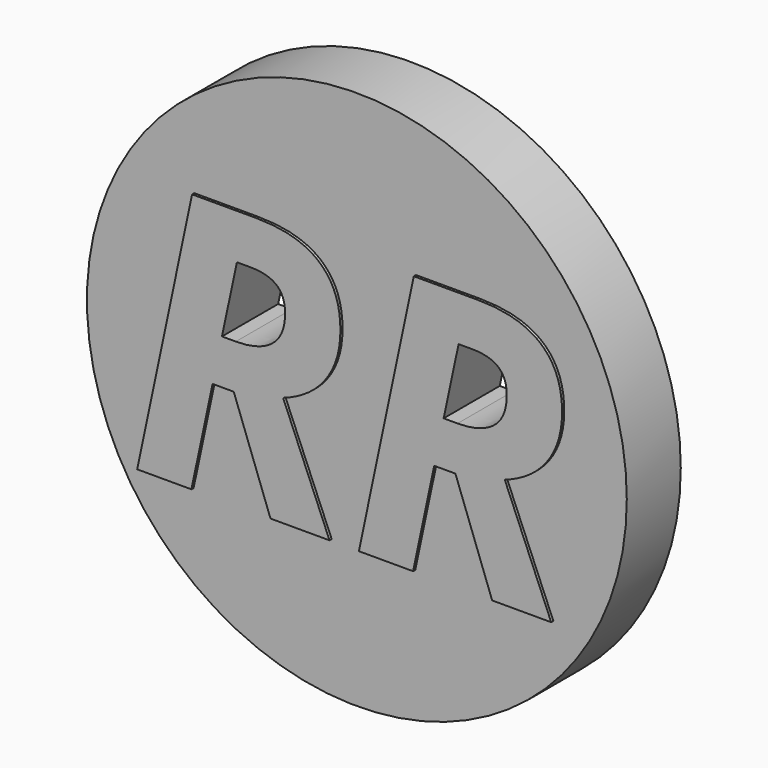
from build123d import *

# Parameters (mm, degrees)
F0_R     = 25.4
F1_DEPTH = 6.35
F3_DEPTH = 6.604
F4_DEPTH = 6.604


# Not quite as in the source:
# - the program builds the solid bodies; features that only make, move or delete a surface that nothing else refers to are left out


with BuildPart() as f1:
    # F0 (on Front) → F1 (new body)
    with BuildSketch(Plane.XZ):
        Circle(F0_R)
        with BuildLine():
            Line((-11.384175581, -2.9492764653), (-13.375339268, -2.9492764653))
            Line((-13.375339268, -2.9492764653), (-15.3665029551, -12.3323677108))
            Line((-15.3665029551, -12.3323677108), (-20.4675217554, -12.3323677108))
            Line((-20.4675217554, -12.3323677108), (-15.3022718684, 12.1236185417))
            Line((-15.3022718684, 12.1236185417), (-9.296665264, 12.1236185417))
            add(Edge.make_bspline(
                [(-9.296665264, 12.1236185417), (-5.3303956617, 12.1236185417), (-3.3392319747, 10.4161421542)],
                knots=[0, 0, 0, 1, 1, 1], degree=2))
            add(Edge.make_bspline(
                [(-3.3392319747, 10.4161421542), (-1.3480682877, 8.7086657667), (-1.3480682877, 5.4168225745)],
                knots=[0, 0, 0, 1, 1, 1], degree=2))
            add(Edge.make_bspline(
                [(-1.3480682877, 5.4168225745), (-1.3480682877, 2.7726428396), (-2.7370655371, 0.8751494873)],
                knots=[0, 0, 0, 1, 1, 1], degree=2))
            add(Edge.make_bspline(
                [(-2.7370655371, 0.8751494873), (-4.1260627865, -1.022343865), (-6.738126978, -1.9429894407)],
                knots=[0, 0, 0, 1, 1, 1], degree=2))
            Line((-6.738126978, -1.9429894407), (-2.370413084, -12.3323677108))
            Line((-2.370413084, -12.3323677108), (-7.9264020816, -12.3323677108))
            Line((-7.9264020816, -12.3323677108), (-11.384175581, -2.9492764653))
        make_face(mode=Mode.SUBTRACT)
        with BuildLine():
            Line((9.4748698175, -2.9492764653), (7.4837061305, -2.9492764653))
            Line((7.4837061305, -2.9492764653), (5.4925424435, -12.3323677108))
            Line((5.4925424435, -12.3323677108), (0.3915236432, -12.3323677108))
            Line((0.3915236432, -12.3323677108), (5.5567735302, 12.1236185417))
            Line((5.5567735302, 12.1236185417), (11.5623801345, 12.1236185417))
            add(Edge.make_bspline(
                [(11.5623801345, 12.1236185417), (15.5286497369, 12.1236185417), (17.5198134239, 10.4161421542)],
                knots=[0, 0, 0, 1, 1, 1], degree=2))
            add(Edge.make_bspline(
                [(17.5198134239, 10.4161421542), (19.5109771109, 8.7086657667), (19.5109771109, 5.4168225745)],
                knots=[0, 0, 0, 1, 1, 1], degree=2))
            add(Edge.make_bspline(
                [(19.5109771109, 5.4168225745), (19.5109771109, 2.7726428396), (18.1219798615, 0.8751494873)],
                knots=[0, 0, 0, 1, 1, 1], degree=2))
            add(Edge.make_bspline(
                [(18.1219798615, 0.8751494873), (16.7329826121, -1.022343865), (14.1209184205, -1.9429894407)],
                knots=[0, 0, 0, 1, 1, 1], degree=2))
            Line((14.1209184205, -1.9429894407), (18.4886323146, -12.3323677108))
            Line((18.4886323146, -12.3323677108), (12.932643317, -12.3323677108))
            Line((12.932643317, -12.3323677108), (9.4748698175, -2.9492764653))
        make_face(mode=Mode.SUBTRACT)
    extrude(amount=F1_DEPTH)

    # F0 (on Front) → F3 (join)
    with BuildSketch(Plane.XZ):
        with BuildLine():
            Line((5.4925424435, -12.3323677108), (7.4837061305, -2.9492764653))
            Line((7.4837061305, -2.9492764653), (9.4748698175, -2.9492764653))
            Line((9.4748698175, -2.9492764653), (12.932643317, -12.3323677108))
            Line((12.932643317, -12.3323677108), (18.4886323146, -12.3323677108))
            Line((18.4886323146, -12.3323677108), (14.1209184205, -1.9429894407))
            add(Edge.make_bspline(
                [(18.1219798615, 0.8751494873), (16.7329826121, -1.022343865), (14.1209184205, -1.9429894407)],
                knots=[0, 0, 0, 1, 1, 1], degree=2))
            add(Edge.make_bspline(
                [(19.5109771109, 5.4168225745), (19.5109771109, 2.7726428396), (18.1219798615, 0.8751494873)],
                knots=[0, 0, 0, 1, 1, 1], degree=2))
            add(Edge.make_bspline(
                [(17.5198134239, 10.4161421542), (19.5109771109, 8.7086657667), (19.5109771109, 5.4168225745)],
                knots=[0, 0, 0, 1, 1, 1], degree=2))
            add(Edge.make_bspline(
                [(11.5623801345, 12.1236185417), (15.5286497369, 12.1236185417), (17.5198134239, 10.4161421542)],
                knots=[0, 0, 0, 1, 1, 1], degree=2))
            Line((11.5623801345, 12.1236185417), (5.5567735302, 12.1236185417))
            Line((5.5567735302, 12.1236185417), (0.3915236432, -12.3323677108))
            Line((0.3915236432, -12.3323677108), (5.4925424435, -12.3323677108))
        make_face()
        with BuildLine():
            Line((9.6729156681, 1.2685648932), (8.3668835723, 1.2685648932))
            Line((8.3668835723, 1.2685648932), (9.7746148887, 7.8736616399))
            Line((9.7746148887, 7.8736616399), (11.0110633072, 7.8736616399))
            add(Edge.make_bspline(
                [(13.5133993923, 7.1885300487), (12.7185396947, 7.8736616399), (11.0110633072, 7.8736616399)],
                knots=[0, 0, 0, 1, 1, 1], degree=2))
            add(Edge.make_bspline(
                [(14.30825909, 5.133135275), (14.30825909, 6.5033984574), (13.5133993923, 7.1885300487)],
                knots=[0, 0, 0, 1, 1, 1], degree=2))
            add(Edge.make_bspline(
                [(13.0851921478, 2.2213260123), (14.30825909, 3.1740871313), (14.30825909, 5.133135275)],
                knots=[0, 0, 0, 1, 1, 1], degree=2))
            add(Edge.make_bspline(
                [(9.6729156681, 1.2685648932), (11.8621252057, 1.2685648932), (13.0851921478, 2.2213260123)],
                knots=[0, 0, 0, 1, 1, 1], degree=2))
        make_face(mode=Mode.SUBTRACT)
    extrude(amount=F3_DEPTH)

    # F0 (on Front) → F4 (join)
    with BuildSketch(Plane.XZ):
        with BuildLine():
            Line((-15.3665029551, -12.3323677108), (-13.375339268, -2.9492764653))
            Line((-13.375339268, -2.9492764653), (-11.384175581, -2.9492764653))
            Line((-11.384175581, -2.9492764653), (-7.9264020816, -12.3323677108))
            Line((-7.9264020816, -12.3323677108), (-2.370413084, -12.3323677108))
            Line((-2.370413084, -12.3323677108), (-6.738126978, -1.9429894407))
            add(Edge.make_bspline(
                [(-2.7370655371, 0.8751494873), (-4.1260627865, -1.022343865), (-6.738126978, -1.9429894407)],
                knots=[0, 0, 0, 1, 1, 1], degree=2))
            add(Edge.make_bspline(
                [(-1.3480682877, 5.4168225745), (-1.3480682877, 2.7726428396), (-2.7370655371, 0.8751494873)],
                knots=[0, 0, 0, 1, 1, 1], degree=2))
            add(Edge.make_bspline(
                [(-3.3392319747, 10.4161421542), (-1.3480682877, 8.7086657667), (-1.3480682877, 5.4168225745)],
                knots=[0, 0, 0, 1, 1, 1], degree=2))
            add(Edge.make_bspline(
                [(-9.296665264, 12.1236185417), (-5.3303956617, 12.1236185417), (-3.3392319747, 10.4161421542)],
                knots=[0, 0, 0, 1, 1, 1], degree=2))
            Line((-9.296665264, 12.1236185417), (-15.3022718684, 12.1236185417))
            Line((-15.3022718684, 12.1236185417), (-20.4675217554, -12.3323677108))
            Line((-20.4675217554, -12.3323677108), (-15.3665029551, -12.3323677108))
        make_face()
        with BuildLine():
            Line((-11.1861297305, 1.2685648932), (-12.4921618262, 1.2685648932))
            Line((-12.4921618262, 1.2685648932), (-11.0844305099, 7.8736616399))
            Line((-11.0844305099, 7.8736616399), (-9.8479820913, 7.8736616399))
            add(Edge.make_bspline(
                [(-7.3456460062, 7.1885300487), (-8.1405057038, 7.8736616399), (-9.8479820913, 7.8736616399)],
                knots=[0, 0, 0, 1, 1, 1], degree=2))
            add(Edge.make_bspline(
                [(-6.5507863086, 5.133135275), (-6.5507863086, 6.5033984574), (-7.3456460062, 7.1885300487)],
                knots=[0, 0, 0, 1, 1, 1], degree=2))
            add(Edge.make_bspline(
                [(-7.7738532507, 2.2213260123), (-6.5507863086, 3.1740871313), (-6.5507863086, 5.133135275)],
                knots=[0, 0, 0, 1, 1, 1], degree=2))
            add(Edge.make_bspline(
                [(-11.1861297305, 1.2685648932), (-8.9969201929, 1.2685648932), (-7.7738532507, 2.2213260123)],
                knots=[0, 0, 0, 1, 1, 1], degree=2))
        make_face(mode=Mode.SUBTRACT)
    extrude(amount=F4_DEPTH)


solid = f1.part
